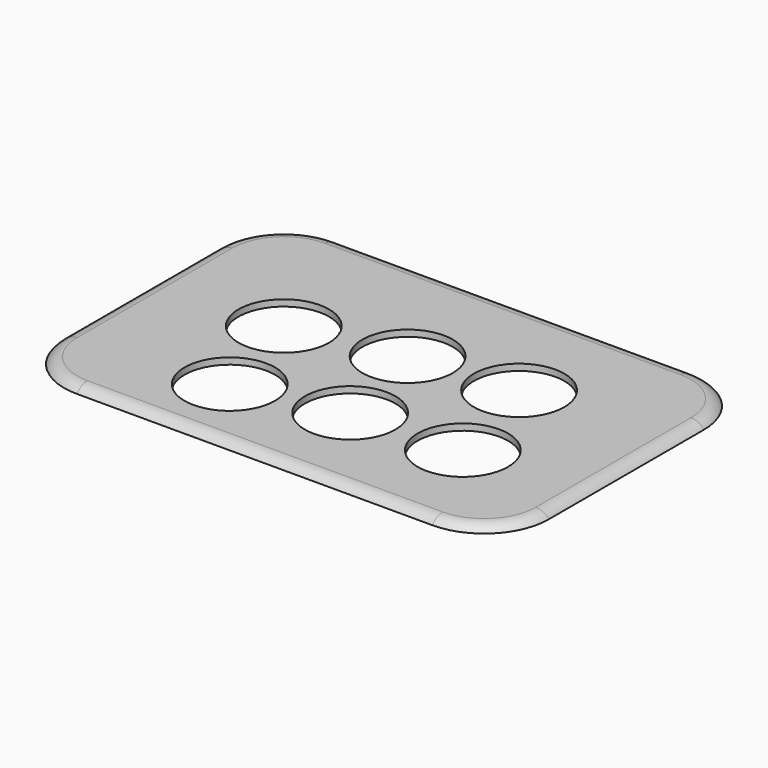
from build123d import *

# Parameters (mm, degrees)
F0_W         = 150
F0_H         = 100
F0_R         = 14
F1_DEPTH     = 2
F2_R         = 20
F3_T1_DEPTH  = 110
F3_T3_DEPTH  = 60
F3_T6_ANGLE  = 90
F3_T8_ANGLE  = 90
F3_T10_ANGLE = 90
F3_T12_ANGLE = 90


# Not quite as in the source:
# - a fillet or chamfer that OpenCascade refuses, or shapes differently, is made with other operations: its cross-section is extruded or revolved along the edge and cut away or added


with BuildPart() as f1:
    # F0 (on Top) → F1 (new body)
    with BuildSketch(Plane.XY):
        Rectangle(F0_W, F0_H)
        with Locations((-27.0043395302, -25.9092412172)):
            Circle(F0_R, mode=Mode.SUBTRACT)
        with Locations((5.1257033043, -19.4994347856)):
            Circle(F0_R, mode=Mode.SUBTRACT)
        with Locations((38.5656639238, -17.7100679294)):
            Circle(F0_R, mode=Mode.SUBTRACT)
        with Locations((-35.8011273407, 5.9865840333)):
            Circle(F0_R, mode=Mode.SUBTRACT)
        with Locations((-2.5469161856, 12.3156928879)):
            Circle(F0_R, mode=Mode.SUBTRACT)
        with Locations((29.6401518762, 15.2098077585)):
            Circle(F0_R, mode=Mode.SUBTRACT)
    extrude(amount=F1_DEPTH)

    # F2
    f2_edges = [f1.edges().sort_by_distance(p)[0] for p in [
        (-75, -50, 1),
        (75, -50, 1),
        (-75, 50, 1),
        (75, 50, 1),
    ]]
    fillet(f2_edges, radius=F2_R)

    # F3: fillet of radius 5 on 2 edges, made by hand

    # F3_s2 → F3_t1 (cut)
    with BuildSketch(Plane.YZ.offset(-55)):
        with BuildLine():
            ThreePointArc((-50, 0), (-48.2360679775, 1.472135955), (-46, 2))
            Line((-46, 2), (-50, 2))
            Line((-50, 2), (-50, 0))
        make_face()
        with BuildLine():
            ThreePointArc((46, 2), (48.2360679775, 1.472135955), (50, 0))
            Line((50, 0), (50, 2))
            Line((50, 2), (46, 2))
        make_face()
    extrude(amount=F3_T1_DEPTH, mode=Mode.SUBTRACT)

    # F3_s4 → F3_t3 (cut)
    with BuildSketch(Plane.XZ.offset(-30)):
        with BuildLine():
            ThreePointArc((-71, 2), (-73.2360679775, 1.472135955), (-75, 0))
            Line((-75, 0), (-75, 2))
            Line((-75, 2), (-71, 2))
        make_face()
        with BuildLine():
            ThreePointArc((71, 2), (73.2360679775, 1.472135955), (75, 0))
            Line((75, 0), (75, 2))
            Line((75, 2), (71, 2))
        make_face()
    extrude(amount=F3_T3_DEPTH, mode=Mode.SUBTRACT)

    # F3_s5 → F3_t6 (revolve, cut)
    with BuildSketch(Plane.YZ.offset(-55)):
        with BuildLine():
            ThreePointArc((-50, 0), (-48.2360679775, 1.472135955), (-46, 2))
            Line((-46, 2), (-50, 2))
            Line((-50, 2), (-50, 0))
        make_face()
    revolve(axis=Axis((-55, -30, 2), (0, 0, -1)), revolution_arc=F3_T6_ANGLE, mode=Mode.SUBTRACT)

    # F3_s7 → F3_t8 (revolve, cut)
    with BuildSketch(Plane.YZ.offset(-55)):
        with BuildLine():
            ThreePointArc((46, 2), (48.2360679775, 1.472135955), (50, 0))
            Line((50, 0), (50, 2))
            Line((50, 2), (46, 2))
        make_face()
    revolve(axis=Axis((-55, 30, 2), (0, 0, 1)), revolution_arc=F3_T8_ANGLE, mode=Mode.SUBTRACT)

    # F3_s9 → F3_t10 (revolve, cut)
    with BuildSketch(Plane.XZ.offset(-30)):
        with BuildLine():
            ThreePointArc((71, 2), (73.2360679775, 1.472135955), (75, 0))
            Line((75, 0), (75, 2))
            Line((75, 2), (71, 2))
        make_face()
    revolve(axis=Axis((55, 30, 2), (0, 0, 1)), revolution_arc=F3_T10_ANGLE, mode=Mode.SUBTRACT)

    # F3_s11 → F3_t12 (revolve, cut)
    with BuildSketch(Plane.YZ.offset(55)):
        with BuildLine():
            ThreePointArc((-50, 0), (-48.2360679775, 1.472135955), (-46, 2))
            Line((-46, 2), (-50, 2))
            Line((-50, 2), (-50, 0))
        make_face()
    revolve(axis=Axis((55, -30, 2), (0, 0, 1)), revolution_arc=F3_T12_ANGLE, mode=Mode.SUBTRACT)


solid = f1.part
